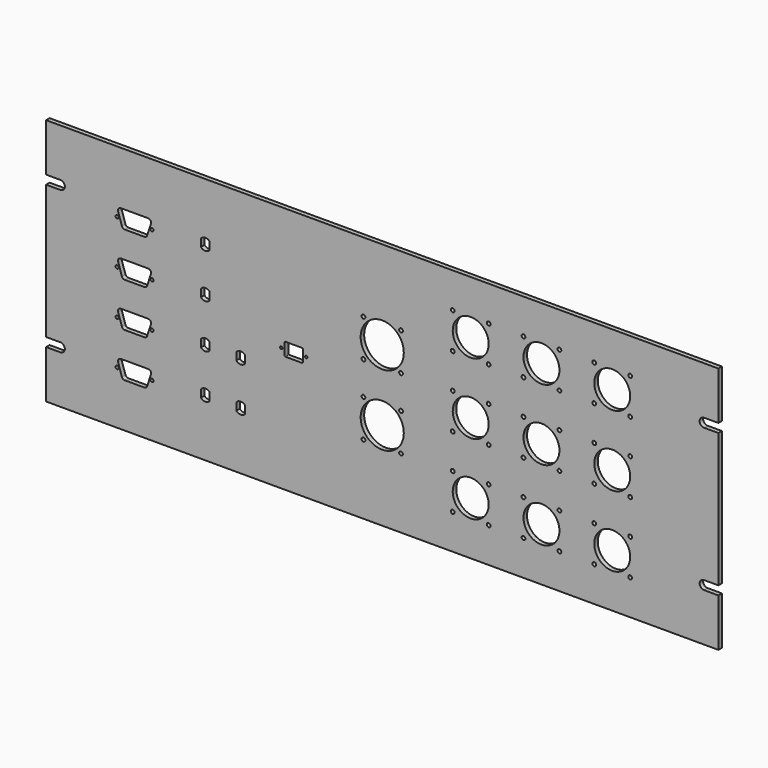
from build123d import *

# Parameters (mm, degrees)
F0_R     = 15.4813
F1_DEPTH = 3.175
F2_D     = 2.7051
F3_D     = 2.2606
F4_D     = 1.778
F5_D     = 2.7051


with BuildPart() as f1:
    # F0 (on Front) → F1 (new body)
    with BuildSketch(Plane.XZ):
        with BuildLine():
            Line((-256.0487464639, -118.0957335805), (-256.0487464639, -152.5127335805))
            Line((-256.0487464639, -152.5127335805), (226.5512535361, -152.5127335805))
            Line((226.5512535361, -152.5127335805), (226.5512535361, -118.0957335805))
            Line((226.5512535361, -118.0957335805), (216.2642535361, -118.0957335805))
            ThreePointArc((216.2642535361, -118.0957335805), (213.0892535361, -114.9207335805), (216.2642535361, -111.7457335805))
            Line((216.2642535361, -111.7457335805), (226.5512535361, -111.7457335805))
            Line((226.5512535361, -111.7457335805), (226.5512535361, -15.4797335805))
            Line((226.5512535361, -15.4797335805), (216.2642535361, -15.4797335805))
            ThreePointArc((216.2642535361, -15.4797335805), (213.0892535361, -12.3047335805), (216.2642535361, -9.1297335805))
            Line((216.2642535361, -9.1297335805), (226.5512535361, -9.1297335805))
            Line((226.5512535361, -9.1297335805), (226.5512535361, 25.2872664195))
            Line((226.5512535361, 25.2872664195), (-256.0487464639, 25.2872664195))
            Line((-256.0487464639, 25.2872664195), (-256.0487464639, -9.1297335805))
            Line((-256.0487464639, -9.1297335805), (-245.7617464639, -9.1297335805))
            ThreePointArc((-245.7617464639, -9.1297335805), (-242.5867464639, -12.3047335805), (-245.7617464639, -15.4797335805))
            Line((-245.7617464639, -15.4797335805), (-256.0487464639, -15.4797335805))
            Line((-256.0487464639, -15.4797335805), (-256.0487464639, -111.7457335805))
            Line((-256.0487464639, -111.7457335805), (-245.7617464639, -111.7457335805))
            ThreePointArc((-245.7617464639, -111.7457335805), (-242.5867464639, -114.9207335805), (-245.7617464639, -118.0957335805))
            Line((-245.7617464639, -118.0957335805), (-256.0487464639, -118.0957335805))
        make_face()
        with BuildLine():
            Line((-201.6108901792, -119.2556428345), (-204.333221176, -110.8720428345))
            ThreePointArc((-204.333221176, -110.8720428345), (-204.033545034, -108.9816114451), (-202.3280867717, -108.1127335805))
            Line((-202.3280867717, -108.1127335805), (-182.769406156, -108.1127335805))
            ThreePointArc((-182.769406156, -108.1127335805), (-181.0639478937, -108.9816114451), (-180.7642717517, -110.8720428345))
            Line((-180.7642717517, -110.8720428345), (-183.4866027485, -119.2556428345))
            ThreePointArc((-183.4866027485, -119.2556428345), (-184.2524150174, -120.3099918428), (-185.4917371528, -120.7127335805))
            Line((-185.4917371528, -120.7127335805), (-199.6057557749, -120.7127335805))
            ThreePointArc((-199.6057557749, -120.7127335805), (-200.8450779104, -120.3099918428), (-201.6108901792, -119.2556428345))
        make_face(mode=Mode.SUBTRACT)
        with BuildLine():
            ThreePointArc((-144.9237464639, -108.5411434448), (-141.7487464639, -107.0721335805), (-138.5737464639, -108.5411434448))
            Line((-138.5737464639, -108.5411434448), (-138.5737464639, -113.9343237162))
            ThreePointArc((-138.5737464639, -113.9343237162), (-141.7487464639, -115.4033335805), (-144.9237464639, -113.9343237162))
            Line((-144.9237464639, -113.9343237162), (-144.9237464639, -108.5411434448))
        make_face(mode=Mode.SUBTRACT)
        with BuildLine():
            ThreePointArc((-119.5237464639, -108.5411434448), (-116.3487464639, -107.0721335805), (-113.1737464639, -108.5411434448))
            Line((-113.1737464639, -108.5411434448), (-113.1737464639, -113.9343237162))
            ThreePointArc((-113.1737464639, -113.9343237162), (-116.3487464639, -115.4033335805), (-119.5237464639, -113.9343237162))
            Line((-119.5237464639, -113.9343237162), (-119.5237464639, -108.5411434448))
        make_face(mode=Mode.SUBTRACT)
        with BuildLine():
            Line((-185.4917371528, -88.9627335805), (-199.6057557749, -88.9627335805))
            ThreePointArc((-199.6057557749, -88.9627335805), (-200.8450779104, -88.5599918428), (-201.6108901792, -87.5056428345))
            Line((-201.6108901792, -87.5056428345), (-204.333221176, -79.1220428345))
            ThreePointArc((-204.333221176, -79.1220428345), (-204.033545034, -77.2316114451), (-202.3280867717, -76.3627335805))
            Line((-202.3280867717, -76.3627335805), (-182.769406156, -76.3627335805))
            ThreePointArc((-182.769406156, -76.3627335805), (-181.0639478937, -77.2316114451), (-180.7642717517, -79.1220428345))
            Line((-180.7642717517, -79.1220428345), (-183.4866027485, -87.5056428345))
            ThreePointArc((-183.4866027485, -87.5056428345), (-184.2524150174, -88.5599918428), (-185.4917371528, -88.9627335805))
        make_face(mode=Mode.SUBTRACT)
        with BuildLine():
            ThreePointArc((-144.9237464639, -76.7911434448), (-141.7487464639, -75.3221335805), (-138.5737464639, -76.7911434448))
            Line((-138.5737464639, -76.7911434448), (-138.5737464639, -82.1843237162))
            ThreePointArc((-138.5737464639, -82.1843237162), (-141.7487464639, -83.6533335805), (-144.9237464639, -82.1843237162))
            Line((-144.9237464639, -82.1843237162), (-144.9237464639, -76.7911434448))
        make_face(mode=Mode.SUBTRACT)
        with Locations((-14.7487464639, -89.0127335805)):
            Circle(F0_R, mode=Mode.SUBTRACT)
        with BuildLine():
            ThreePointArc((-119.5237464639, -76.7911434448), (-116.3487464639, -75.3221335805), (-113.1737464639, -76.7911434448))
            Line((-113.1737464639, -76.7911434448), (-113.1737464639, -82.1843237162))
            ThreePointArc((-113.1737464639, -82.1843237162), (-116.3487464639, -83.6533335805), (-119.5237464639, -82.1843237162))
            Line((-119.5237464639, -82.1843237162), (-119.5237464639, -76.7911434448))
        make_face(mode=Mode.SUBTRACT)
        with BuildLine():
            ThreePointArc((48.7512535361, -127.3159335805), (35.8480535361, -114.4127335805), (48.7512535361, -101.5095335805))
            ThreePointArc((48.7512535361, -101.5095335805), (61.6544535361, -114.4127335805), (48.7512535361, -127.3159335805))
        make_face(mode=Mode.SUBTRACT)
        with BuildLine():
            ThreePointArc((99.5512535361, -127.3159335805), (86.6480535361, -114.4127335805), (99.5512535361, -101.5095335805))
            ThreePointArc((99.5512535361, -101.5095335805), (112.4544535361, -114.4127335805), (99.5512535361, -127.3159335805))
        make_face(mode=Mode.SUBTRACT)
        with BuildLine():
            ThreePointArc((150.3512535361, -127.3159335805), (137.4480535361, -114.4127335805), (150.3512535361, -101.5095335805))
            ThreePointArc((150.3512535361, -101.5095335805), (163.2544535361, -114.4127335805), (150.3512535361, -127.3159335805))
        make_face(mode=Mode.SUBTRACT)
        with BuildLine():
            Line((-185.4917371528, -57.2127335805), (-199.6057557749, -57.2127335805))
            ThreePointArc((-199.6057557749, -57.2127335805), (-200.8450779104, -56.8099918428), (-201.6108901792, -55.7556428345))
            Line((-201.6108901792, -55.7556428345), (-204.333221176, -47.3720428345))
            ThreePointArc((-204.333221176, -47.3720428345), (-204.033545034, -45.4816114451), (-202.3280867717, -44.6127335805))
            Line((-202.3280867717, -44.6127335805), (-182.769406156, -44.6127335805))
            ThreePointArc((-182.769406156, -44.6127335805), (-181.0639478937, -45.4816114451), (-180.7642717517, -47.3720428345))
            Line((-180.7642717517, -47.3720428345), (-183.4866027485, -55.7556428345))
            ThreePointArc((-183.4866027485, -55.7556428345), (-184.2524150174, -56.8099918428), (-185.4917371528, -57.2127335805))
        make_face(mode=Mode.SUBTRACT)
        with BuildLine():
            ThreePointArc((-144.9237464639, -45.0411434448), (-141.7487464639, -43.5721335805), (-138.5737464639, -45.0411434448))
            Line((-138.5737464639, -45.0411434448), (-138.5737464639, -50.4343237162))
            ThreePointArc((-138.5737464639, -50.4343237162), (-141.7487464639, -51.9033335805), (-144.9237464639, -50.4343237162))
            Line((-144.9237464639, -50.4343237162), (-144.9237464639, -45.0411434448))
        make_face(mode=Mode.SUBTRACT)
        with BuildLine():
            Line((-185.4917371528, -25.4627335805), (-199.6057557749, -25.4627335805))
            ThreePointArc((-199.6057557749, -25.4627335805), (-200.8450779104, -25.0599918428), (-201.6108901792, -24.0056428345))
            Line((-201.6108901792, -24.0056428345), (-204.333221176, -15.6220428345))
            ThreePointArc((-204.333221176, -15.6220428345), (-204.033545034, -13.7316114451), (-202.3280867717, -12.8627335805))
            Line((-202.3280867717, -12.8627335805), (-182.769406156, -12.8627335805))
            ThreePointArc((-182.769406156, -12.8627335805), (-181.0639478937, -13.7316114451), (-180.7642717517, -15.6220428345))
            Line((-180.7642717517, -15.6220428345), (-183.4866027485, -24.0056428345))
            ThreePointArc((-183.4866027485, -24.0056428345), (-184.2524150174, -25.0599918428), (-185.4917371528, -25.4627335805))
        make_face(mode=Mode.SUBTRACT)
        with BuildLine():
            ThreePointArc((-71.7463464639, -67.8545335805), (-71.895136219, -68.2137438253), (-72.2543464639, -68.3625335805))
            Line((-72.2543464639, -68.3625335805), (-84.2431464639, -68.3625335805))
            ThreePointArc((-84.2431464639, -68.3625335805), (-84.6023567087, -68.2137438253), (-84.7511464639, -67.8545335805))
            Line((-84.7511464639, -67.8545335805), (-84.7511464639, -59.3709335805))
            ThreePointArc((-84.7511464639, -59.3709335805), (-84.6023567087, -59.0117233357), (-84.2431464639, -58.8629335805))
            Line((-84.2431464639, -58.8629335805), (-72.2543464639, -58.8629335805))
            ThreePointArc((-72.2543464639, -58.8629335805), (-71.895136219, -59.0117233357), (-71.7463464639, -59.3709335805))
            Line((-71.7463464639, -59.3709335805), (-71.7463464639, -67.8545335805))
        make_face(mode=Mode.SUBTRACT)
        with Locations((-14.7487464639, -38.2127335805)):
            Circle(F0_R, mode=Mode.SUBTRACT)
        with BuildLine():
            ThreePointArc((-144.9237464639, -13.2911434448), (-141.7487464639, -11.8221335805), (-138.5737464639, -13.2911434448))
            Line((-138.5737464639, -13.2911434448), (-138.5737464639, -18.6843237162))
            ThreePointArc((-138.5737464639, -18.6843237162), (-141.7487464639, -20.1533335805), (-144.9237464639, -18.6843237162))
            Line((-144.9237464639, -18.6843237162), (-144.9237464639, -13.2911434448))
        make_face(mode=Mode.SUBTRACT)
        with BuildLine():
            ThreePointArc((48.7512535361, -76.5159335805), (35.8480535361, -63.6127335805), (48.7512535361, -50.7095335805))
            ThreePointArc((48.7512535361, -50.7095335805), (61.6544535361, -63.6127335805), (48.7512535361, -76.5159335805))
        make_face(mode=Mode.SUBTRACT)
        with BuildLine():
            ThreePointArc((99.5512535361, -76.5159335805), (86.6480535361, -63.6127335805), (99.5512535361, -50.7095335805))
            ThreePointArc((99.5512535361, -50.7095335805), (112.4544535361, -63.6127335805), (99.5512535361, -76.5159335805))
        make_face(mode=Mode.SUBTRACT)
        with BuildLine():
            ThreePointArc((150.3512535361, -76.5159335805), (137.4480535361, -63.6127335805), (150.3512535361, -50.7095335805))
            ThreePointArc((150.3512535361, -50.7095335805), (163.2544535361, -63.6127335805), (150.3512535361, -76.5159335805))
        make_face(mode=Mode.SUBTRACT)
        with BuildLine():
            ThreePointArc((48.7512535361, -25.7159335805), (35.8480535361, -12.8127335805), (48.7512535361, 0.0904664195))
            ThreePointArc((48.7512535361, 0.0904664195), (61.6544535361, -12.8127335805), (48.7512535361, -25.7159335805))
        make_face(mode=Mode.SUBTRACT)
        with BuildLine():
            ThreePointArc((99.5512535361, -25.7159335805), (86.6480535361, -12.8127335805), (99.5512535361, 0.0904664195))
            ThreePointArc((99.5512535361, 0.0904664195), (112.4544535361, -12.8127335805), (99.5512535361, -25.7159335805))
        make_face(mode=Mode.SUBTRACT)
        with BuildLine():
            ThreePointArc((150.3512535361, -25.7159335805), (137.4480535361, -12.8127335805), (150.3512535361, 0.0904664195))
            ThreePointArc((150.3512535361, 0.0904664195), (163.2544535361, -12.8127335805), (150.3512535361, -25.7159335805))
        make_face(mode=Mode.SUBTRACT)
    extrude(amount=F1_DEPTH)

    # F2 (through all)
    with Locations(Plane(origin=(0, 0, 0), x_dir=(1, 0, 0), z_dir=(0, 1, 0))):
        with Locations((35.8544035361, -0.0841164195), (61.6481035361, -0.0841164195), (61.6481035361, 25.7095835805), (35.8544035361, 25.7095835805), (86.6544035361, 25.7095835805), (112.4481035361, 25.7095835805), (112.4481035361, -0.0841164195), (86.6544035361, -0.0841164195), (35.8544035361, 50.7158835805), (61.6481035361, 50.7158835805), (86.6544035361, 50.7158835805), (112.4481035361, 50.7158835805), (137.4544035361, -0.0841164195), (163.2481035361, -0.0841164195), (163.2481035361, 25.7095835805), (137.4544035361, 25.7095835805), (137.4544035361, 50.7158835805), (163.2481035361, 50.7158835805), (35.8544035361, 76.5095835805), (61.6481035361, 76.5095835805), (86.6544035361, 76.5095835805), (112.4481035361, 76.5095835805), (137.4544035361, 76.5095835805), (163.2481035361, 76.5095835805), (163.2481035361, 101.5158835805), (137.4544035361, 101.5158835805), (112.4481035361, 101.5158835805), (86.6544035361, 101.5158835805), (61.6481035361, 101.5158835805), (35.8544035361, 101.5158835805), (35.8544035361, 127.3095835805), (61.6481035361, 127.3095835805), (86.6544035361, 127.3095835805), (112.4481035361, 127.3095835805), (137.4544035361, 127.3095835805), (163.2481035361, 127.3095835805)):
            Hole(F2_D / 2)

    # F3 (through all)
    with Locations(Plane(origin=(0, 0, 0), x_dir=(1, 0, 0), z_dir=(0, 1, 0))):
        with Locations((-180.0519464639, 114.4127335805), (-205.0455464639, 114.4127335805), (-205.0455464639, 82.6627335805), (-180.0519464639, 82.6627335805), (-180.0519464639, 50.9127335805), (-205.0455464639, 50.9127335805), (-205.0455464639, 19.1627335805), (-180.0519464639, 19.1627335805)):
            Hole(F3_D / 2)

    # F4 (through all)
    with Locations(Plane(origin=(0, 0, 0), x_dir=(1, 0, 0), z_dir=(0, 1, 0))):
        with Locations((-69.2444464639, 63.6127335805), (-87.2530464639, 63.6127335805)):
            Hole(F4_D / 2)

    # F5 (through all)
    with Locations(Plane(origin=(0, 0, 0), x_dir=(1, 0, 0), z_dir=(0, 1, 0))):
        with Locations((-1.2613464639, 24.7253335805), (-28.2361464639, 24.7253335805), (-28.2361464639, 51.7001335805), (-1.2613464639, 51.7001335805), (-28.2361464639, 75.5253335805), (-1.2613464639, 75.5253335805), (-1.2613464639, 102.5001335805), (-28.2361464639, 102.5001335805)):
            Hole(F5_D / 2)


solid = f1.part
